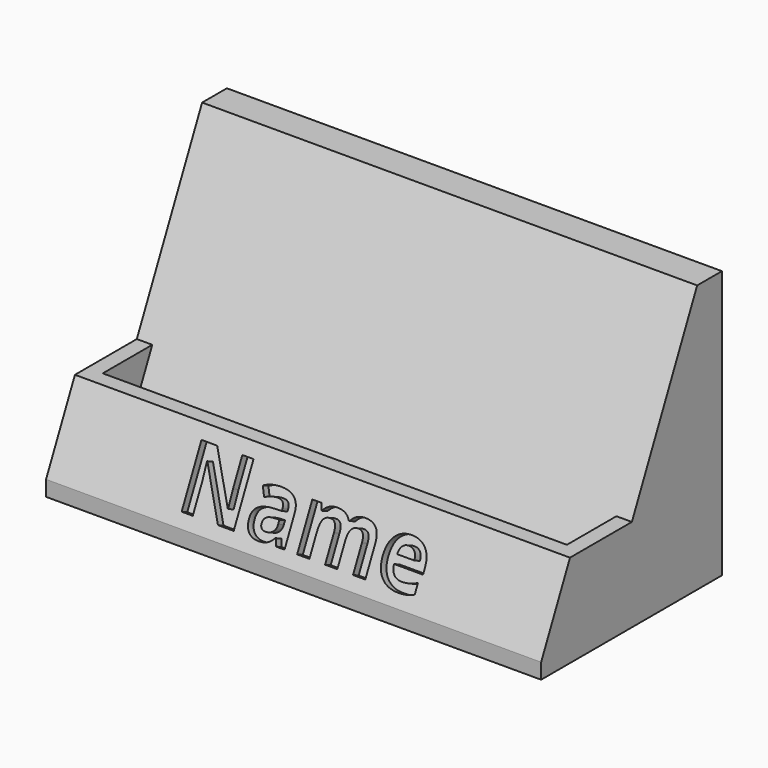
from build123d import *

# Parameters (mm, degrees)
F1_DEPTH     = 47.625
F3_DEPTH     = 3.175
F5_DEPTH     = 3.175
F6_TEXT_SIZE = 16.8683200166
F7_DEPTH     = 1.5875


# Not quite as in the source:
# - Text() gives the source's letters only with a copy of the font that has no kerning and outlines rounded to 1/6400 em; it was checked with that copy


with BuildPart() as f1:
    # F0 (on Right) → F1 (new body, symmetric)
    with BuildSketch(Plane.YZ):
        Polygon((0, 3.175), (0, 0), (46.3776336585, 0), (46.3776336585, 54.9704900291), (40.0276336585, 54.9704900291), (15.875, 3.175), (3.175, 3.175), (10.5776340732, 19.05), (7.4026340732, 19.05), align=None)
        Polygon((19.3782248927, 3.175), (42.0503317365, 51.7954900291), (43.2026336585, 51.7954900291), (43.2026336585, 3.175), align=None, mode=Mode.SUBTRACT)
    extrude(amount=F1_DEPTH, both=True)

    # F2 (on face) → F3 (join)
    with BuildSketch(Plane.YZ.offset(47.625)):
        Polygon((23.2776340732, 19.05), (7.4026340732, 19.05), (0, 3.175), (0, 0), (46.3776336585, 0), (46.3776336585, 54.9704900291), (40.0276336585, 54.9704900291), align=None)
    extrude(amount=F3_DEPTH)

    # F4 (on face) → F5 (join)
    with BuildSketch(Plane(origin=(-47.625, 0, 0), x_dir=(0, -1, 0), z_dir=(-1, 0, 0))):
        Polygon((0, 3.175), (-7.4026340732, 19.05), (-23.2776340732, 19.05), (-40.0276336585, 54.9704900291), (-46.3776336585, 54.9704900291), (-46.3776336585, 0), (0, 0), align=None)
    extrude(amount=F5_DEPTH)

    # F6 (on face) → F7 (cut)
    with BuildSketch(Plane(origin=(0, -1.2160955535, 0.5670746696), x_dir=(1, 0, 0), z_dir=(0, -0.906307787, 0.4226182617))):
        with Locations((-25.4, 5.5629942496)):
            Text('Name', F6_TEXT_SIZE, font='Open Sans', font_style=FontStyle.BOLD, text_align=(TextAlign.LEFT, TextAlign.BOTTOM))
    extrude(amount=-F7_DEPTH, mode=Mode.SUBTRACT)


solid = f1.part
